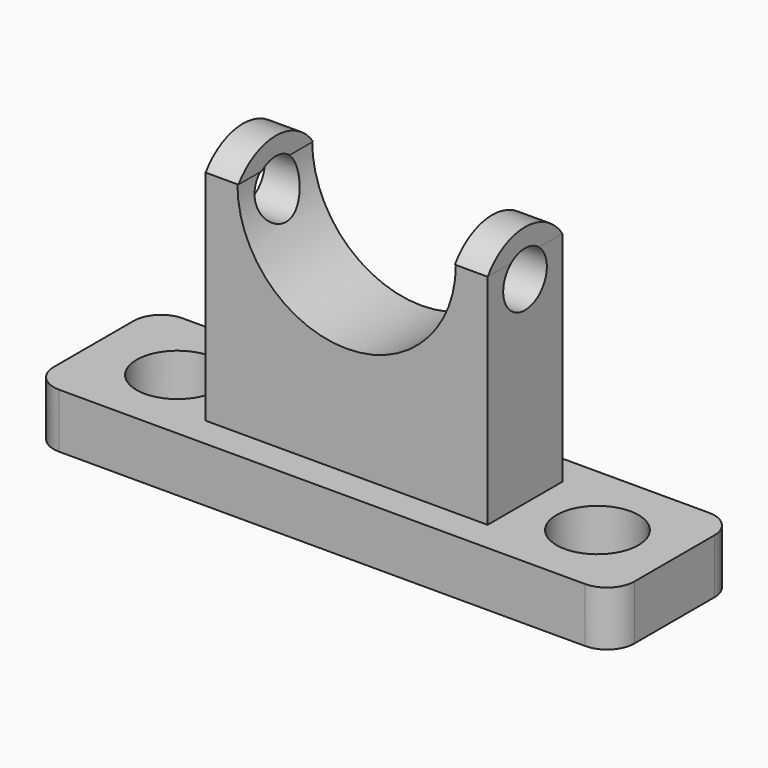
from build123d import *

# Parameters (mm, degrees)
F1_DEPTH    = 12.7
F2_W        = 65.5919536948
F2_H        = 21.728605032
F3_DEPTH    = 50.8
F5_D        = 50.8
F7_DEPTH    = 7.62
F9_DEPTH    = 7.62
F11_D       = 19.05
F13_D       = 19.05
F15_D       = 12.7
F15_DEPTH   = 100.3181093762
F15_2_D     = 12.7
F15_2_DEPTH = 100.3181093762


with BuildPart() as f1:
    # F0 (on Top) → F1 (new body)
    with BuildSketch(Plane.XY):
        with BuildLine():
            ThreePointArc((67.5211325288, 11.6217894644), (65.6612605893, 16.1119175249), (61.1711325288, 17.9717894644))
            Line((61.1711325288, 17.9717894644), (-61.1711325288, 17.9717894644))
            ThreePointArc((-61.1711325288, 17.9717894644), (-65.6612605893, 16.1119175249), (-67.5211325288, 11.6217894644))
            Line((-67.5211325288, 11.6217894644), (-67.5211325288, -11.6217894644))
            ThreePointArc((-67.5211325288, -11.6217894644), (-65.6612605893, -16.1119175249), (-61.1711325288, -17.9717894644))
            Line((-61.1711325288, -17.9717894644), (61.1711325288, -17.9717894644))
            ThreePointArc((61.1711325288, -17.9717894644), (65.6612605893, -16.1119175249), (67.5211325288, -11.6217894644))
            Line((67.5211325288, -11.6217894644), (67.5211325288, 11.6217894644))
        make_face()
    extrude(amount=F1_DEPTH)

    # F2 (on face) → F3 (join)
    with BuildSketch(Plane.XY.offset(12.7)):
        Rectangle(F2_W, F2_H)
    extrude(amount=F3_DEPTH)

    # F5 (through all)
    with Locations(Plane.XZ.offset(10.864302516)):
        with Locations((0, 63.5)):
            Hole(F5_D / 2)

    # F6 (on face) → F7 (join)
    with BuildSketch(Plane(origin=(-32.7959768474, 0, 0), x_dir=(0, -1, 0), z_dir=(-1, 0, 0))):
        with BuildLine():
            Line((-10.864302516, 63.5), (10.864302516, 63.5))
            ThreePointArc((10.864302516, 63.5), (0, 69.114496873), (-10.864302516, 63.5))
        make_face()
    extrude(amount=-F7_DEPTH)

    # F11 (through all)
    with Locations(Plane.XY.offset(12.7)):
        with Locations((-48.0263084173, 0)):
            Hole(F11_D / 2)

    # F13 (through all)
    with Locations(Plane.XY.offset(12.7)):
        with Locations((49.6508777142, 0)):
            Hole(F13_D / 2)

    # F15 (through all, one way)
    with BuildSketch(Plane(origin=(-32.7959768474, 0, 0), x_dir=(0, -1, 0), z_dir=(-1, 0, 0))):
        with Locations((0, 58.5860051215)):
            Circle(F15_D / 2)
    extrude(amount=-F15_DEPTH, mode=Mode.SUBTRACT)


with BuildPart() as f9:
    # F8 (on face) → F9 (new body)
    with BuildSketch(Plane.YZ.offset(32.7959768474)):
        with BuildLine():
            Line((-10.864302516, 63.5), (10.864302516, 63.5))
            ThreePointArc((10.864302516, 63.5), (0, 69.2741527548), (-10.864302516, 63.5))
        make_face()
    extrude(amount=-F9_DEPTH)

    # F15#2 (through all, one way)
    with BuildSketch(Plane(origin=(-32.7959768474, 0, 0), x_dir=(0, -1, 0), z_dir=(-1, 0, 0))):
        with Locations((0, 58.5860051215)):
            Circle(F15_2_D / 2)
    extrude(amount=-F15_2_DEPTH, mode=Mode.SUBTRACT)


solid = Compound([f1.part, f9.part])
